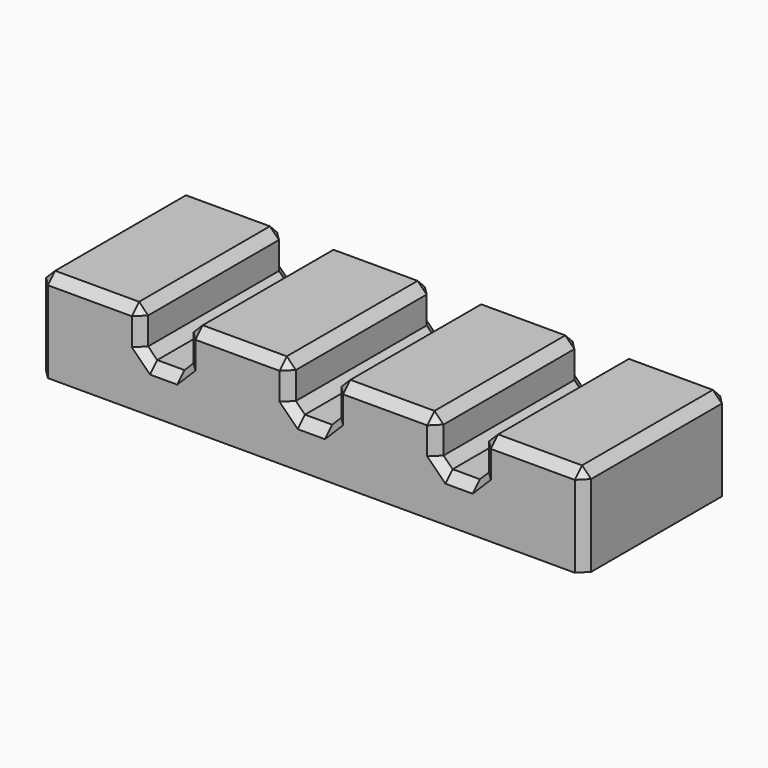
from build123d import *

# Parameters (mm, degrees)
F0_W         = 76.2
F0_H         = 25.4
F1_DEPTH     = 12.7
F2_W         = 6.35
F2_H         = 12.7
F3_DEPTH     = 25.401
F4_SIZE      = 1.27
F5_T         = 2.54
F5_T3_DEPTH  = 6.8760512242
F5_T5_DEPTH  = 6.8760512242
F5_T7_DEPTH  = 6.8760512242
F5_T9_DEPTH  = 6.8760512242
F5_T11_DEPTH = 6.8760512242
F5_T13_DEPTH = 6.8760512242
F5_T15_DEPTH = 6.8760512242
F5_T17_DEPTH = 27.94
F5_T19_DEPTH = 6.8760512242
F5_T21_DEPTH = 6.8760512242
F5_T23_DEPTH = 6.8760512242
F5_T25_DEPTH = 6.8760512242
F5_T27_DEPTH = 6.8760512242
F5_T29_DEPTH = 6.8760512242
F5_T31_DEPTH = 6.8760512242


# Not quite as in the source:
# - a shell that OpenCascade refuses in one call is made with other operations: the cavity is built on its own and cut out


with BuildPart() as f1:
    # F0 (on Top) → F1 (new body)
    with BuildSketch(Plane.XY):
        Rectangle(F0_W, F0_H)
    extrude(amount=F1_DEPTH)

    # F2 (on face) → F3 (cut, through all)
    with BuildSketch(Plane.XZ.offset(12.7)):
        with Locations((0, 12.7)):
            Rectangle(F2_W, F2_H)
        with Locations((20.6502, 12.7)):
            Rectangle(F2_W, F2_H)
        with Locations((-20.6502, 12.7)):
            Rectangle(F2_W, F2_H)
    extrude(amount=-F3_DEPTH, mode=Mode.SUBTRACT)

    # F4
    f4_edges = [f1.edges().sort_by_distance(p)[0] for p in [
        (-23.8252, 0, 12.7),
        (-30.9626, -12.7, 12.7),
        (-38.1, 0, 12.7),
        (-30.9626, 12.7, 12.7),
        (-3.175, 0, 12.7),
        (-10.3251, -12.7, 12.7),
        (-17.4752, 0, 12.7),
        (-10.3251, 12.7, 12.7),
        (17.4752, 0, 12.7),
        (10.3251, -12.7, 12.7),
        (3.175, 0, 12.7),
        (10.3251, 12.7, 12.7),
        (38.1, 0, 12.7),
        (30.9626, -12.7, 12.7),
        (23.8252, 0, 12.7),
        (30.9626, 12.7, 12.7),
        (-20.6502, -12.7, 6.35),
        (-17.4752, 0, 6.35),
        (-20.6502, 12.7, 6.35),
        (-23.8252, 0, 6.35),
        (0, -12.7, 6.35),
        (3.175, 0, 6.35),
        (0, 12.7, 6.35),
        (-3.175, 0, 6.35),
        (20.6502, -12.7, 6.35),
        (23.8252, 0, 6.35),
        (20.6502, 12.7, 6.35),
        (17.4752, 0, 6.35),
        (-38.1, -12.7, 6.35),
        (38.1, -12.7, 6.35),
        (38.1, 12.7, 6.35),
        (-38.1, 12.7, 6.35),
        (-23.8252, 12.7, 9.525),
        (-17.4752, 12.7, 9.525),
        (-3.175, 12.7, 9.525),
        (3.175, 12.7, 9.525),
        (17.4752, 12.7, 9.525),
        (23.8252, 12.7, 9.525),
        (-23.8252, -12.7, 9.525),
        (-17.4752, -12.7, 9.525),
        (-3.175, -12.7, 9.525),
        (3.175, -12.7, 9.525),
        (17.4752, -12.7, 9.525),
        (23.8252, -12.7, 9.525),
    ]]
    chamfer(f4_edges, length=F4_SIZE)

    # F5: shell of thickness 2.54, made by hand


with BuildPart() as f5_core1:
    # F5_t2: copy of F1
    add(f1.part)

    # the walls: a layer under each face that stays
    f5_faces = [f5_core1.faces().sort_by_distance(p)[0] for p in [
        (24.5533333333, 12.7, 5.715),
        (37.465, 12.065, 5.715),
        (-37.465, 12.065, 5.715),
        (30.9626, 12.065, 12.065),
        (-30.9626, 12.065, 12.065),
        (24.4602, 12.065, 9.525),
        (-24.4602, 12.065, 9.525),
        (23.5077, 12.065, 6.6675),
        (-23.5077, 12.065, 6.6675),
        (20.6502, 12.065, 5.715),
        (-20.6502, 12.065, 5.715),
        (17.7927, 12.065, 6.6675),
        (-17.7927, 12.065, 6.6675),
        (16.8402, 12.065, 9.525),
        (-16.8402, 12.065, 9.525),
        (10.3251, 12.065, 12.065),
        (-10.3251, 12.065, 12.065),
        (3.81, 12.065, 9.525),
        (-3.81, 12.065, 9.525),
        (2.8575, 12.065, 6.6675),
        (-2.8575, 12.065, 6.6675),
        (0, 12.065, 5.715),
        (38.1, 0, 5.715),
        (-38.1, 0, 5.715),
        (37.465, -12.065, 5.715),
        (-37.465, -12.065, 5.715),
        (-24.5533333333, -12.7, 5.715),
        (37.1475, 12.065, 11.7475),
        (-37.1475, 12.065, 11.7475),
        (30.9626, 0, 12.7),
        (24.7777, 12.065, 11.7475),
        (-24.7777, 12.065, 11.7475),
        (-30.9626, 0, 12.7),
        (23.8252, 0, 9.525),
        (-23.8252, 0, 9.525),
        (23.1902, 0, 6.985),
        (-23.1902, 0, 6.985),
        (20.6502, 0, 6.35),
        (-20.6502, 0, 6.35),
        (18.1102, 0, 6.985),
        (-18.1102, 0, 6.985),
        (16.5227, 12.065, 11.7475),
        (17.4752, 0, 9.525),
        (-17.4752, 0, 9.525),
        (-16.5227, 12.065, 11.7475),
        (10.3251, 0, 12.7),
        (4.1275, 12.065, 11.7475),
        (-4.1275, 12.065, 11.7475),
        (-10.3251, 0, 12.7),
        (3.175, 0, 9.525),
        (-3.175, 0, 9.525),
        (2.54, 0, 6.985),
        (-2.54, 0, 6.985),
        (0, 0, 6.35),
        (37.465, 0, 12.065),
        (-37.465, 0, 12.065),
        (37.1475, -12.065, 11.7475),
        (-37.465, -11.7475, 11.7475),
        (-30.9626, -12.065, 12.065),
        (30.9626, -12.065, 12.065),
        (-24.4602, -12.065, 9.525),
        (24.4602, -12.065, 9.525),
        (-23.5077, -12.065, 6.6675),
        (23.5077, -12.065, 6.6675),
        (-20.6502, -12.065, 5.715),
        (20.6502, -12.065, 5.715),
        (-17.7927, -12.065, 6.6675),
        (17.7927, -12.065, 6.6675),
        (-16.8402, -12.065, 9.525),
        (16.8402, -12.065, 9.525),
        (-10.3251, -12.065, 12.065),
        (10.3251, -12.065, 12.065),
        (-3.81, -12.065, 9.525),
        (3.81, -12.065, 9.525),
        (-2.8575, -12.065, 6.6675),
        (2.8575, -12.065, 6.6675),
        (0, -12.065, 5.715),
        (24.4602, 0, 12.065),
        (-24.4602, 0, 12.065),
        (16.8402, 0, 12.065),
        (-16.8402, 0, 12.065),
        (3.81, 0, 12.065),
        (-3.81, 0, 12.065),
        (-24.7777, -12.065, 11.7475),
        (24.4602, -11.7475, 11.7475),
        (-16.8402, -11.7475, 11.7475),
        (16.5227, -12.065, 11.7475),
        (-4.1275, -12.065, 11.7475),
        (3.81, -11.7475, 11.7475),
    ]]
    thicken(f5_faces, amount=-F5_T, mode=Mode.SUBTRACT)

    # F5_s4 → F5_t3 (cut)
    with BuildSketch(Plane(origin=(20.6936512242, 20.6936512242, 0), x_dir=(0, 0, 1), z_dir=(-0.7071067812, -0.7071067812, 0))):
        Polygon((7.6346646968, -8.718590961), (7.62, -11.3047299742), (6.8126933972, -11.3047299742), (6.1535303163, -10.8386312897), align=None)
    extrude(amount=F5_T3_DEPTH, mode=Mode.SUBTRACT)

    # F5_s6 → F5_t5 (cut)
    with BuildSketch(Plane(origin=(-20.6936512242, 20.6936512242, 0), x_dir=(0, 0, 1), z_dir=(0.7071067812, -0.7071067812, 0))):
        Polygon((7.6346646968, 8.718590961), (7.62, 11.3047299742), (6.8126933972, 11.3047299742), (6.1535303163, 10.8386312897), align=None)
    extrude(amount=F5_T5_DEPTH, mode=Mode.SUBTRACT)

    # F5_s8 → F5_t7 (cut)
    with BuildSketch(Plane(origin=(0, 5.6060512242, -5.6060512242), x_dir=(1, 0, 0), z_dir=(0, -0.7071067812, 0.7071067812))):
        Polygon((22.5405353032, 12.6184975827), (24.0216696837, 10.4984572539), (23.3625066028, 10.0323585695), (22.5552, 10.0323585695), align=None)
        Polygon((-22.5405353032, 12.6184975827), (-24.0216696837, 10.4984572539), (-23.3625066028, 10.0323585695), (-22.5552, 10.0323585695), align=None)
        Polygon((18.7598646968, 12.6184975827), (18.7452, 10.0323585695), (17.9378933972, 10.0323585695), (17.2787303163, 10.4984572539), align=None)
        Polygon((-18.7598646968, 12.6184975827), (-18.7452, 10.0323585695), (-17.9378933972, 10.0323585695), (-17.2787303163, 10.4984572539), align=None)
        Polygon((1.8903353032, 12.6184975827), (3.3714696837, 10.4984572539), (2.7123066028, 10.0323585695), (1.905, 10.0323585695), align=None)
        Polygon((-1.8903353032, 12.6184975827), (-3.3714696837, 10.4984572539), (-2.7123066028, 10.0323585695), (-1.905, 10.0323585695), align=None)
    extrude(amount=F5_T7_DEPTH, mode=Mode.SUBTRACT)

    # F5_s10 → F5_t9 (cut)
    with BuildSketch(Plane(origin=(-0.0434512242, 0.0434512242, 0), x_dir=(0, 0, 1), z_dir=(0.7071067812, -0.7071067812, 0))):
        Polygon((7.6346646968, -20.4852019447), (6.1535303163, -18.365161616), (6.8126933972, -17.8990629316), (7.62, -17.8990629316), align=None)
    extrude(amount=F5_T9_DEPTH, mode=Mode.SUBTRACT)

    # F5_s12 → F5_t11 (cut)
    with BuildSketch(Plane(origin=(0.0434512242, 0.0434512242, 0), x_dir=(0, 0, 1), z_dir=(-0.7071067812, -0.7071067812, 0))):
        Polygon((7.6346646968, 20.4852019447), (6.1535303163, 18.365161616), (6.8126933972, 17.8990629316), (7.62, 17.8990629316), align=None)
    extrude(amount=F5_T11_DEPTH, mode=Mode.SUBTRACT)

    # F5_s14 → F5_t13 (cut)
    with BuildSketch(Plane(origin=(10.3685512242, 10.3685512242, 0), x_dir=(0, 0, 1), z_dir=(-0.7071067812, -0.7071067812, 0))):
        Polygon((7.6346646968, 5.8833054919), (7.62, 3.2971664787), (6.8126933972, 3.2971664787), (6.1535303163, 3.7632651631), align=None)
    extrude(amount=F5_T13_DEPTH, mode=Mode.SUBTRACT)

    # F5_s16 → F5_t15 (cut)
    with BuildSketch(Plane(origin=(-10.3685512242, 10.3685512242, 0), x_dir=(0, 0, 1), z_dir=(0.7071067812, -0.7071067812, 0))):
        Polygon((7.6346646968, -5.8833054919), (7.62, -3.2971664787), (6.8126933972, -3.2971664787), (6.1535303163, -3.7632651631), align=None)
    extrude(amount=F5_T15_DEPTH, mode=Mode.SUBTRACT)

    # F5_s18 → F5_t17 (cut)
    with BuildSketch(Plane.XZ.offset(-13.97)):
        Polygon((23.7818394878, 7.6379605122), (26.3652, 7.62), (26.3652, 6.5678975516), (25.6212512242, 5.8239487758), align=None)
        Polygon((-23.7818394878, 7.6379605122), (-26.3652, 7.62), (-26.3652, 6.5678975516), (-25.6212512242, 5.8239487758), align=None)
        Polygon((22.5372394878, 6.3933605122), (24.3512512242, 4.5539487758), (23.6073024484, 3.81), (22.5552, 3.81), align=None)
        Polygon((-22.5372394878, 6.3933605122), (-24.3512512242, 4.5539487758), (-23.6073024484, 3.81), (-22.5552, 3.81), align=None)
        Polygon((18.7631605122, 6.3933605122), (18.7452, 3.81), (17.6930975516, 3.81), (16.9491487758, 4.5539487758), align=None)
        Polygon((-18.7631605122, 6.3933605122), (-18.7452, 3.81), (-17.6930975516, 3.81), (-16.9491487758, 4.5539487758), align=None)
        Polygon((17.5185605122, 7.6379605122), (15.6791487758, 5.8239487758), (14.9352, 6.5678975516), (14.9352, 7.62), align=None)
        Polygon((-17.5185605122, 7.6379605122), (-15.6791487758, 5.8239487758), (-14.9352, 6.5678975516), (-14.9352, 7.62), align=None)
        Polygon((3.1316394878, 7.6379605122), (5.715, 7.62), (5.715, 6.5678975516), (4.9710512242, 5.8239487758), align=None)
        Polygon((-3.1316394878, 7.6379605122), (-5.715, 7.62), (-5.715, 6.5678975516), (-4.9710512242, 5.8239487758), align=None)
        Polygon((1.8870394878, 6.3933605122), (3.7010512242, 4.5539487758), (2.9571024484, 3.81), (1.905, 3.81), align=None)
        Polygon((-1.8870394878, 6.3933605122), (-3.7010512242, 4.5539487758), (-2.9571024484, 3.81), (-1.905, 3.81), align=None)
    extrude(amount=F5_T17_DEPTH, mode=Mode.SUBTRACT)

    # F5_s20 → F5_t19 (cut)
    with BuildSketch(Plane(origin=(-20.6936512242, -20.6936512242, 0), x_dir=(0, 0, 1), z_dir=(0.7071067812, 0.7071067812, 0))):
        Polygon((7.6346646968, -8.718590961), (7.62, -11.3047299742), (6.8126933972, -11.3047299742), (6.1535303163, -10.8386312897), align=None)
    extrude(amount=F5_T19_DEPTH, mode=Mode.SUBTRACT)

    # F5_s22 → F5_t21 (cut)
    with BuildSketch(Plane(origin=(20.6936512242, -20.6936512242, 0), x_dir=(0, 0, 1), z_dir=(-0.7071067812, 0.7071067812, 0))):
        Polygon((7.6346646968, 8.718590961), (7.62, 11.3047299742), (6.8126933972, 11.3047299742), (6.1535303163, 10.8386312897), align=None)
    extrude(amount=F5_T21_DEPTH, mode=Mode.SUBTRACT)

    # F5_s24 → F5_t23 (cut)
    with BuildSketch(Plane(origin=(0, -5.6060512242, -5.6060512242), x_dir=(1, 0, 0), z_dir=(0, 0.7071067812, 0.7071067812))):
        Polygon((-22.5405353032, -12.6184975827), (-24.0216696837, -10.4984572539), (-23.3625066028, -10.0323585695), (-22.5552, -10.0323585695), align=None)
        Polygon((22.5405353032, -12.6184975827), (24.0216696837, -10.4984572539), (23.3625066028, -10.0323585695), (22.5552, -10.0323585695), align=None)
        Polygon((-18.7598646968, -12.6184975827), (-18.7452, -10.0323585695), (-17.9378933972, -10.0323585695), (-17.2787303163, -10.4984572539), align=None)
        Polygon((18.7598646968, -12.6184975827), (18.7452, -10.0323585695), (17.9378933972, -10.0323585695), (17.2787303163, -10.4984572539), align=None)
        Polygon((-1.8903353032, -12.6184975827), (-3.3714696837, -10.4984572539), (-2.7123066028, -10.0323585695), (-1.905, -10.0323585695), align=None)
        Polygon((1.8903353032, -12.6184975827), (3.3714696837, -10.4984572539), (2.7123066028, -10.0323585695), (1.905, -10.0323585695), align=None)
    extrude(amount=F5_T23_DEPTH, mode=Mode.SUBTRACT)

    # F5_s26 → F5_t25 (cut)
    with BuildSketch(Plane(origin=(0.0434512242, -0.0434512242, 0), x_dir=(0, 0, 1), z_dir=(-0.7071067812, 0.7071067812, 0))):
        Polygon((7.6346646968, -20.4852019447), (6.1535303163, -18.365161616), (6.8126933972, -17.8990629316), (7.62, -17.8990629316), align=None)
    extrude(amount=F5_T25_DEPTH, mode=Mode.SUBTRACT)

    # F5_s28 → F5_t27 (cut)
    with BuildSketch(Plane(origin=(-0.0434512242, -0.0434512242, 0), x_dir=(0, 0, 1), z_dir=(0.7071067812, 0.7071067812, 0))):
        Polygon((7.6346646968, 20.4852019447), (6.1535303163, 18.365161616), (6.8126933972, 17.8990629316), (7.62, 17.8990629316), align=None)
    extrude(amount=F5_T27_DEPTH, mode=Mode.SUBTRACT)

    # F5_s30 → F5_t29 (cut)
    with BuildSketch(Plane(origin=(-10.3685512242, -10.3685512242, 0), x_dir=(0, 0, 1), z_dir=(0.7071067812, 0.7071067812, 0))):
        Polygon((7.6346646968, 5.8833054919), (7.62, 3.2971664787), (6.8126933972, 3.2971664787), (6.1535303163, 3.7632651631), align=None)
    extrude(amount=F5_T29_DEPTH, mode=Mode.SUBTRACT)

    # F5_s32 → F5_t31 (cut)
    with BuildSketch(Plane(origin=(10.3685512242, -10.3685512242, 0), x_dir=(0, 0, 1), z_dir=(-0.7071067812, 0.7071067812, 0))):
        Polygon((7.6346646968, -5.8833054919), (7.62, -3.2971664787), (6.8126933972, -3.2971664787), (6.1535303163, -3.7632651631), align=None)
    extrude(amount=F5_T31_DEPTH, mode=Mode.SUBTRACT)


with BuildPart() as f1_1:
    add(f1.part)

    # what is left inside the walls is the cavity
    f5_cavity = [f5_core1.part.solids().sort_by_distance(p)[0] for p in [
        (0, -3.386667, 0.0254),
    ]]
    add(f5_cavity, mode=Mode.SUBTRACT)


solid = f1_1.part
